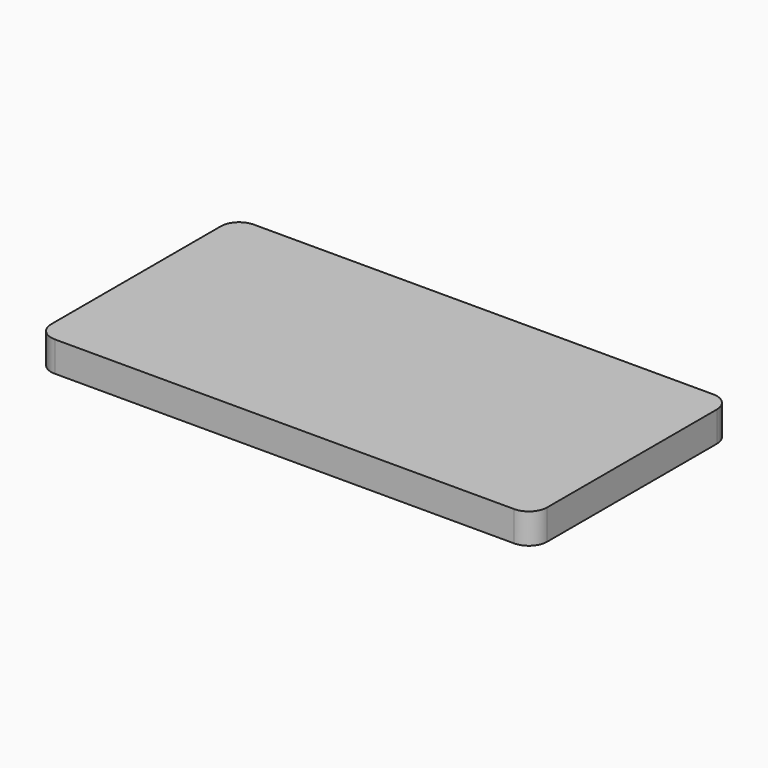
from build123d import *

# Parameters (mm, degrees)
F0_W     = 137.5156
F0_H     = 68.9356
F1_DEPTH = 8.382
F2_R     = 5.08
F3_R     = 6.9215
F4_DEPTH = 1.27
F5_R     = 1.26999


# Not quite as in the source:
# - a fillet or chamfer is up to 0.001 mm smaller than in the source, because OpenCascade refuses the exact size


with BuildPart() as f1:
    # F0 (on Top) → F1 (new body)
    with BuildSketch(Plane.XY):
        Rectangle(F0_W, F0_H)
    extrude(amount=F1_DEPTH)

    # F2
    f2_edges = [f1.edges().sort_by_distance(p)[0] for p in [
        (-68.7578, 34.4678, 4.191),
        (-68.7578, -34.4678, 4.191),
        (68.7578, -34.4678, 4.191),
        (68.7578, 34.4678, 4.191),
    ]]
    fillet(f2_edges, radius=F2_R)

    # F3 (on face) → F4 (join)
    with BuildSketch(Plane(origin=(0, 0, 0), x_dir=(1, 0, 0), z_dir=(0, 0, -1))):
        with Locations((52.1843, 17.8943)):
            Circle(F3_R)
    extrude(amount=F4_DEPTH)

    # F5 (radius 1.27 in the source; OpenCascade refuses exactly that, so slightly less here)
    f5_edges = [f1.edges().sort_by_distance(p)[0] for p in [
        (45.2628, -17.8943, -1.27),
    ]]
    fillet(f5_edges, radius=F5_R)


solid = f1.part
